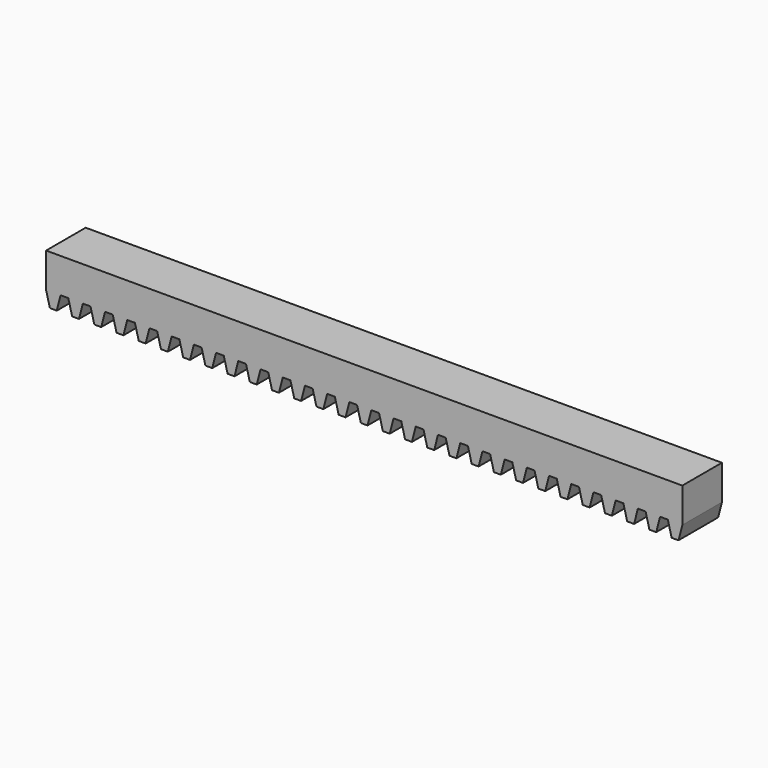
from build123d import *

# Parameters (mm, degrees)
F1_DEPTH = 12.7


# Not quite as in the source:
# - a feature of the source that left no trace in its solid (it failed there, or was rolled back) is left out


with BuildPart() as f1:
    # F0 (on Front) → F1 (new body)
    with BuildSketch(Plane.XZ):
        Polygon((26.4879943687, -2.5616034378), (26.4879943687, 6.35), (-136.7738045981, 6.35), (-136.7738045981, -2.5616034378), (-136.5471367316, -3.4380630457), (-135.7986113058, -6.3323961114), (-134.0326395944, -6.346404838), (-133.0482363701, -2.54), (-131.0740445981, -2.54), (-130.837778613, -3.4535727787), (-130.0892531872, -6.3479058444), (-128.3328795944, -6.3651881602), (-127.3484763701, -2.5587833222), (-125.3742845981, -2.5587833222), (-125.138018613, -3.4723561009), (-124.3938092991, -6.35), (-122.9682044968, -6.35), (-122.6284623376, -6.35), (-121.6487163701, -2.5616034378), (-119.6745245981, -2.5616034378), (-119.438258613, -3.4751762165), (-118.6947786306, -6.35), (-117.8373619914, -6.35), (-117.2674353611, -6.35), (-116.9287023376, -6.35), (-115.9489563701, -2.5616034378), (-113.9747645981, -2.5616034378), (-112.9950186306, -6.35), (-112.1405051147, -6.35), (-111.2289423376, -6.35), (-110.2491963701, -2.5616034378), (-108.2750045981, -2.5616034378), (-107.2952586306, -6.35), (-106.4407451147, -6.35), (-105.5291823376, -6.35), (-104.5494363701, -2.5616034378), (-102.5752445981, -2.5616034378), (-101.5954986306, -6.35), (-100.7409851147, -6.35), (-99.8294223376, -6.35), (-98.8496763701, -2.5616034378), (-96.8754845981, -2.5616034378), (-95.8957386306, -6.35), (-95.0412251147, -6.35), (-94.1296623376, -6.35), (-93.1499163701, -2.5616034378), (-91.1757245981, -2.5616034378), (-90.1959786306, -6.35), (-89.3414651147, -6.35), (-88.4299023376, -6.35), (-87.4501563701, -2.5616034378), (-85.4759645981, -2.5616034378), (-84.4962186306, -6.35), (-82.7252846402, -6.35), (-81.7503963701, -2.58038676), (-79.7762045981, -2.58038676), (-78.801316328, -6.35), (-77.9419451147, -6.35), (-77.0303823376, -6.35), (-76.0506363701, -2.5616034378), (-74.0764445981, -2.5616034378), (-73.0966986306, -6.35), (-72.2421851147, -6.35), (-71.3306223376, -6.35), (-70.3508763701, -2.5616034378), (-68.3766845981, -2.5616034378), (-67.3969386306, -6.35), (-66.5424251147, -6.35), (-65.6308623376, -6.35), (-64.6511163701, -2.5616034378), (-62.6769245981, -2.5616034378), (-61.6971786306, -6.35), (-60.8426651147, -6.35), (-59.9311023376, -6.35), (-58.9513563701, -2.5616034378), (-56.9771645981, -2.5616034378), (-55.9974186306, -6.35), (-54.2883915989, -6.35), (-53.3086456314, -2.5616034378), (-53.2515963701, -2.5616034378), (-51.3344538594, -2.5616034378), (-50.3547078919, -6.35), (-49.4431451147, -6.35), (-48.5886315989, -6.35), (-47.6088856314, -2.5616034378), (-45.6346938594, -2.5616034378), (-44.6549478919, -6.35), (-43.7433851147, -6.35), (-42.8888715989, -6.35), (-41.9091256314, -2.5616034378), (-39.9349338594, -2.5616034378), (-38.9551878919, -6.35), (-38.0436251147, -6.35), (-37.1891115989, -6.35), (-36.2093656314, -2.5616034378), (-34.2351738594, -2.5616034378), (-33.2554278919, -6.35), (-32.3438651147, -6.35), (-31.4844939015, -6.35), (-30.5096056314, -2.58038676), (-28.5354138594, -2.58038676), (-27.5605255893, -6.35), (-25.7895915989, -6.35), (-24.8098456314, -2.5616034378), (-22.8356538594, -2.5616034378), (-21.8559078919, -6.35), (-20.9443451147, -6.35), (-20.0898315989, -6.35), (-19.1100856314, -2.5616034378), (-17.1358938594, -2.5616034378), (-16.1561478919, -6.35), (-15.2445851147, -6.35), (-14.3900715989, -6.35), (-13.4103256314, -2.5616034378), (-11.4361338594, -2.5616034378), (-10.4563878919, -6.35), (-9.5448251147, -6.35), (-8.6903115989, -6.35), (-7.7105656314, -2.5616034378), (-5.7363738594, -2.5616034378), (-4.7566278919, -6.35), (-3.8450651147, -6.35), (-2.9905515989, -6.35), (-2.0108056314, -2.5616034378), (-0.0366138594, -2.5616034378), (0.9431321081, -6.35), (1.8546948853, -6.35), (2.7092084011, -6.35), (3.6889543686, -2.5616034378), (5.6631461406, -2.5616034378), (6.6428921081, -6.35), (8.4089684011, -6.35), (9.3887143686, -2.5616034378), (11.3629061406, -2.5616034378), (12.3426521081, -6.35), (14.1079990696, -6.35), (15.0884743686, -2.5587833222), (17.0626661406, -2.5587833222), (18.0470693649, -6.3651881602), (19.8034429577, -6.3479058444), (20.7882343686, -2.54), (22.7624261406, -2.54), (23.7468293649, -6.346404838), (25.5128010763, -6.3323961114), align=None)
    extrude(amount=-F1_DEPTH)


solid = f1.part
